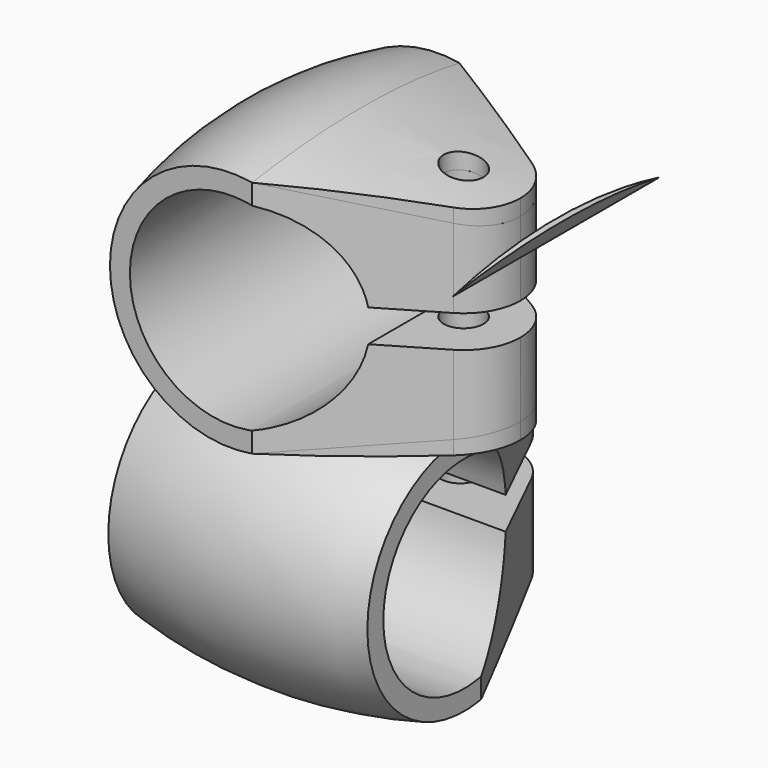
from build123d import *

# Parameters (mm, degrees)
F1_DEPTH  = 16
F5_DEPTH  = 16
F10_START = -25
F9_R      = 2.4522993316
F10_DEPTH = 167.5566196442
F12_R     = 2.4522993316
F13_DEPTH = 195.4795867205


with BuildPart() as f1:
    # F0 (on Right) → F1 (new body, symmetric)
    with BuildSketch(Plane.YZ):
        with BuildLine():
            Line((27.3389626793, 2), (27.3389626793, 7.8722359036))
            Line((27.3389626793, 7.8722359036), (2.1706022208, 12.3100969127))
            ThreePointArc((2.1706022208, 12.3100969127), (8.8997973564, 8.777448776), (12.3389626793, 2))
            Line((12.3389626793, 2), (27.3389626793, 2))
        make_face()
        with BuildLine():
            Line((27.3389626793, 10.3722359036), (2.5981274, 14.7347126886))
            ThreePointArc((2.5981274, 14.7347126886), (-14.9620193825, 0), (2.5981274, -14.7347126886))
            Line((2.5981274, -14.7347126886), (27.3389626793, -10.3722359036))
            Line((27.3389626793, -10.3722359036), (27.3389626793, -7.8722359036))
            Line((27.3389626793, -7.8722359036), (2.1706022208, -12.3100969127))
            ThreePointArc((2.1706022208, -12.3100969127), (-12.5, 0), (2.1706022208, 12.3100969127))
            Line((2.1706022208, 12.3100969127), (27.3389626793, 7.8722359036))
            Line((27.3389626793, 7.8722359036), (27.3389626793, 10.3722359036))
        make_face()
        with BuildLine():
            Line((2.1706022208, -12.3100969127), (27.3389626793, -7.8722359036))
            Line((27.3389626793, -7.8722359036), (27.3389626793, -2))
            Line((27.3389626793, -2), (12.3389626793, -2))
            ThreePointArc((12.3389626793, -2), (8.8997973564, -8.777448776), (2.1706022208, -12.3100969127))
        make_face()
    extrude(amount=F1_DEPTH, both=True)

    # F3: sweep along a path in F3_path
    with BuildLine(Plane(origin=(16, 27.3389626793, 10.3722359036), x_dir=(0, 0, 1), z_dir=(1, 0, 0))) as f3_path:
        Line((0, 0), (4.362476785, 24.7408352793))
        ThreePointArc((4.362476785, 24.7408352793), (-10.3722359036, 42.3009820618), (-25.1069485923, 24.7408352793))
        Line((-25.1069485923, 24.7408352793), (-20.7444718073, 0))
    # F2 (on face) → F3 (sweep)
    with BuildSketch(Plane(origin=(0, 27.3389626793, 0), x_dir=(-1, 0, 0), z_dir=(0, 1, 0))):
        with BuildLine():
            Line((-16, 10.3722359036), (16, 10.3722359036))
            ThreePointArc((16, 10.3722359036), (0, 12.3722359036), (-16, 10.3722359036))
        make_face()
    sweep(path=f3_path.line)

    # F9 (on offset) → F10 (cut)
    with BuildSketch(Plane(origin=(0, 0, -148), x_dir=(1, 0, 0), z_dir=(0, 0, -1)).offset(F10_START)):
        with BuildLine():
            Line((-16, -2.5981274), (-16, -31.1659335838))
            Line((-16, -31.1659335838), (16, -31.1659335838))
            Line((16, -31.1659335838), (16, -2.5981274))
            Line((16, -2.5981274), (6.2896922875, -22.4765383075))
            ThreePointArc((6.2896922875, -22.4765383075), (0, -26.4041172869), (-6.2896922875, -22.4765383075))
            Line((-6.2896922875, -22.4765383075), (-16, -2.5981274))
        make_face()
        with Locations((0, -19.4041172869)):
            Circle(F9_R)
    extrude(amount=-F10_DEPTH, mode=Mode.SUBTRACT)


with BuildPart() as f5:
    # F4 (on Front) → F5 (new body, symmetric)
    with BuildSketch(Plane.XZ):
        with BuildLine():
            Line((27.3389626793, 31.9240387651), (27.3389626793, 37.7962746687))
            Line((27.3389626793, 37.7962746687), (2.1706022208, 42.2341356777))
            ThreePointArc((2.1706022208, 42.2341356777), (8.8997973564, 38.7014875411), (12.3389626793, 31.9240387651))
            Line((12.3389626793, 31.9240387651), (27.3389626793, 31.9240387651))
        make_face()
        with BuildLine():
            Line((27.3389626793, 40.2962746687), (2.5981274, 44.6587514537))
            ThreePointArc((2.5981274, 44.6587514537), (-14.9620193825, 29.9240387651), (2.5981274, 15.1893260764))
            Line((2.5981274, 15.1893260764), (27.3389626793, 19.5518028614))
            Line((27.3389626793, 19.5518028614), (27.3389626793, 22.0518028614))
            Line((27.3389626793, 22.0518028614), (2.1706022208, 17.6139418524))
            ThreePointArc((2.1706022208, 17.6139418524), (-12.5, 29.9240387651), (2.1706022208, 42.2341356777))
            Line((2.1706022208, 42.2341356777), (27.3389626793, 37.7962746687))
            Line((27.3389626793, 37.7962746687), (27.3389626793, 40.2962746687))
        make_face()
        with BuildLine():
            Line((2.1706022208, 17.6139418524), (27.3389626793, 22.0518028614))
            Line((27.3389626793, 22.0518028614), (27.3389626793, 27.9240387651))
            Line((27.3389626793, 27.9240387651), (12.3389626793, 27.9240387651))
            ThreePointArc((12.3389626793, 27.9240387651), (8.8997973564, 21.1465899891), (2.1706022208, 17.6139418524))
        make_face()
    extrude(amount=F5_DEPTH, both=True)


with BuildPart() as f7:
    # F7: sweep along a path in F7_path
    with BuildLine(Plane(origin=(27.3389626793, -16, 40.2962746687), x_dir=(0, 0, 1), z_dir=(0, -1, 0))) as f7_path:
        Line((0, 0), (4.362476785, 24.7408352793))
        ThreePointArc((4.362476785, 24.7408352793), (-10.3722359036, 42.3009820618), (-25.1069485923, 24.7408352793))
        Line((-25.1069485923, 24.7408352793), (-20.7444718073, 0))
    # F6 (on face) → F7 (sweep)
    with BuildSketch(Plane.YZ.offset(27.3389626793)):
        with BuildLine():
            Line((16, 19.5518028614), (-16, 19.5518028614))
            ThreePointArc((-16, 19.5518028614), (0, 17.5518028614), (16, 19.5518028614))
        make_face()
    sweep(path=f7_path.line)


with BuildPart() as f13_tool:
    # F12 (on offset) → F13 (new body)
    with BuildSketch(Plane.XY.offset(177.9240387651)):
        with BuildLine():
            Line((2.5981274, -16), (27.3389626793, -16))
            Line((27.3389626793, -16), (27.3389626793, 16))
            Line((27.3389626793, 16), (2.5981274, 16))
            Line((2.5981274, 16), (19.4829733323, 6.0272072796))
            ThreePointArc((19.4829733323, 6.0272072796), (22.0025297711, 3.469928937), (22.9230895689, 0))
            ThreePointArc((22.9230895689, 0), (22.0025297711, -3.469928937), (19.4829733323, -6.0272072796))
            Line((19.4829733323, -6.0272072796), (2.5981274, -16))
        make_face()
        with Locations((15.9230895689, 0)):
            Circle(F12_R)
    extrude(amount=-F13_DEPTH)


with BuildPart() as f5_1:
    add(f5.part)

    # F13: cut by f13_tool
    add(f13_tool.part, mode=Mode.SUBTRACT)


with BuildPart() as f7_1:
    add(f7.part)

    # F13: cut by f13_tool
    add(f13_tool.part, mode=Mode.SUBTRACT)


solid = Compound([f1.part, f5_1.part, f7_1.part])
